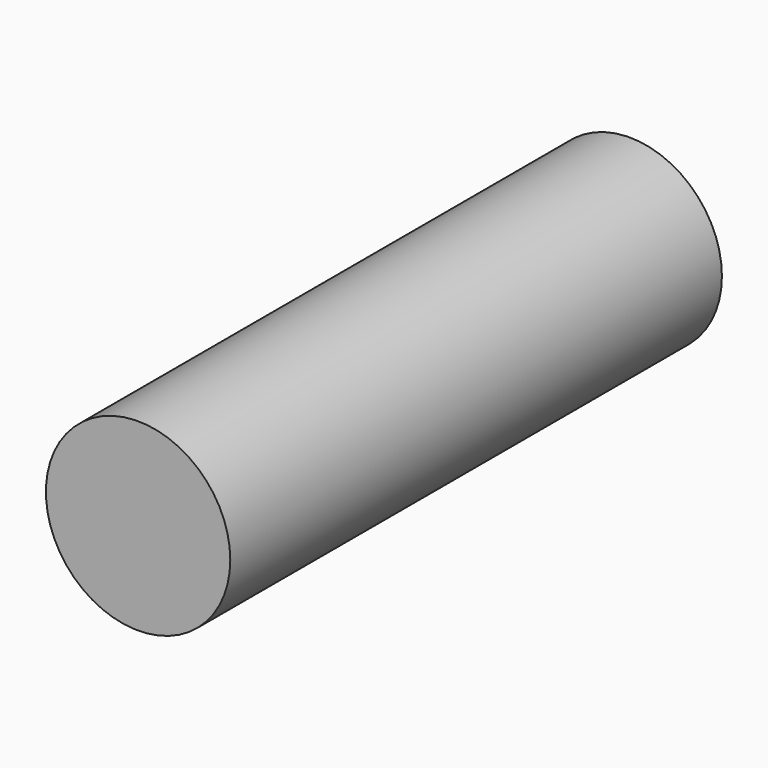
from build123d import *

# Parameters (mm, degrees)
F0_W = 114.3
F0_H = 381


# Not quite as in the source:
# - the program builds the solid bodies; features that only make, move or delete a surface that nothing else refers to are left out


with BuildPart() as f1:
    # F0 (on Top) → F1 (revolve)
    with BuildSketch(Plane.XY):
        with Locations((57.15, 190.5)):
            Rectangle(F0_W, F0_H)
        with Locations((57.15, -190.5)):
            Rectangle(F0_W, F0_H)
    revolve(axis=Axis((0, 0, 0), (0, -1, 0)))


solid = f1.part
